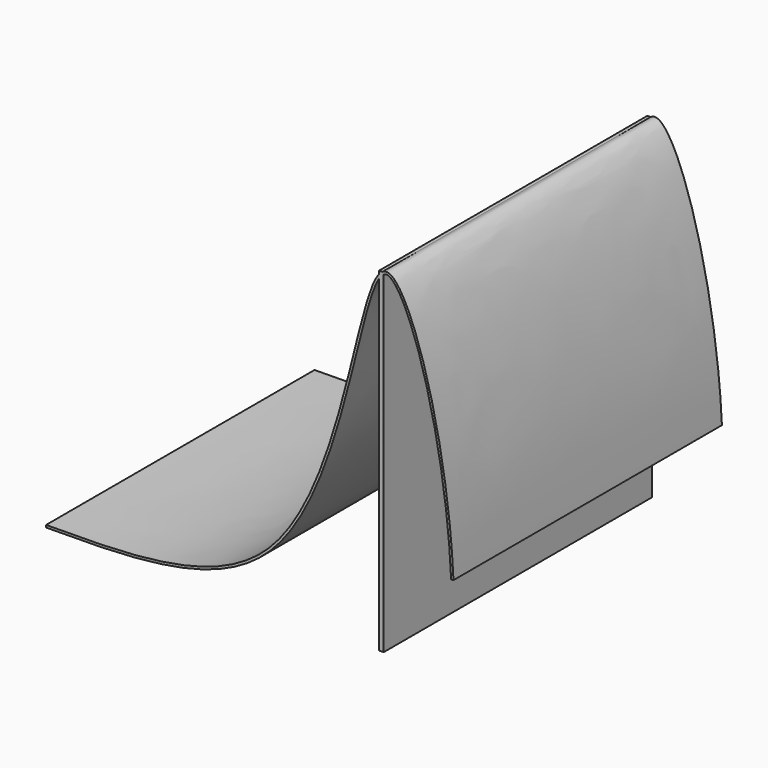
from build123d import *

# Parameters (mm, degrees)
F1_DEPTH = 914.4


# Not quite as in the source:
# - ends of sketch curves that miss each other by under 0.0002 mm in the source are joined
# - the dataset's text gives a spline's control points without its knots; the knots are read off the source's solid


with BuildPart() as f1:
    # F0 (on Front) → F1 (new body)
    with BuildSketch(Plane.XZ):
        with BuildLine():
            add(Edge.make_bspline(
                [(-919.8371731596, 0), (-666.6549326545, 0), (-224.5771125372, 9.857256005), (-90.4120834618, 673.3494347676), (-31.042313376, 873.5728945456), (-12.7, 896.4040661924)],
                knots=[0, 0, 0, 0, 0.2772976129, 0.5617641499, 0.6630198034, 0.6630198034, 0.6630198034, 0.6630198034], degree=3))
            Line((-919.8371731596, 0), (-919.8371731596, -6.35))
            add(Edge.make_bspline(
                [(-919.8371731596, -6.35), (-891.2956817484, -6.35), (-835.0727771699, -6.2264734906), (-753.6955894076, -4.5537616294), (-675.6488494754, -0.2717047035), (-601.3027865804, 7.749478894), (-531.0281070337, 20.6510983897), (-476.1747806697, 36.433071437), (-434.7209643178, 52.6606822547), (-404.9003603349, 66.7779757198), (-376.407262262, 82.9857781471), (-353.8198862803, 98.3520654174), (-336.4752851305, 111.8293289531), (-323.8373430454, 122.5464690045), (-311.5775291009, 133.8876328292), (-299.7039715139, 145.875207016), (-288.2290876414, 158.4866993511), (-273.4422137623, 176.0875345027), (-255.8954652009, 199.4854636313), (-236.2518066429, 229.5516028845), (-211.8312721359, 271.9684188112), (-184.4187186541, 328.7539699263), (-155.8635982627, 401.0055012331), (-131.028728694, 475.4527935567), (-109.3069067738, 550.1778688522), (-90.0991494945, 623.2560938642), (-75.6932560314, 681.1724555189), (-64.8354875196, 724.7427710564), (-56.9528674516, 755.7967634626), (-49.2605256897, 784.9693353051), (-41.6751107234, 811.8671692139), (-34.1167291745, 836.1005454151), (-26.516271345, 857.2638545274), (-20.1072029881, 871.9856586334), (-15.4866518, 880.7508103168), (-13.4472817504, 884.1799958005), (-12.7, 885.3770727094)],
                knots=[0, 0, 0, 0, 0.03125, 0.0625, 0.09375, 0.125, 0.15625, 0.1875, 0.203125, 0.21875, 0.234375, 0.25, 0.2578125, 0.265625, 0.2734375, 0.28125, 0.2890625, 0.296875, 0.3125, 0.328125, 0.34375, 0.375, 0.40625, 0.4375, 0.46875, 0.5, 0.53125, 0.546875, 0.5625, 0.578125, 0.59375, 0.609375, 0.625, 0.640625, 0.6484375, 0.6529650593, 0.6529650593, 0.6529650593, 0.6529650593], degree=3))
            Line((-12.7, 885.3770727094), (-12.7, 896.4040661924))
        make_face()
        with BuildLine():
            Line((-12.7, 904.875), (-12.7, 896.4040661924))
            add(Edge.make_bspline(
                [(-12.7, 896.4040661924), (-9.8289625515, 899.9777238573), (-6.8903732232, 902.823006869), (-3.8687211654, 904.875)],
                knots=[0.6630198034, 0.6630198034, 0.6630198034, 0.6630198034, 0.6788688824, 0.6788688824, 0.6788688824, 0.6788688824], degree=3))
            Line((-3.8687211654, 904.875), (-12.7, 904.875))
        make_face()
        with BuildLine():
            add(Edge.make_bspline(
                [(-12.7, 896.4040661924), (-9.8289625515, 899.9777238573), (-6.8903732232, 902.823006869), (-3.8687211654, 904.875)],
                knots=[0.6630198034, 0.6630198034, 0.6630198034, 0.6630198034, 0.6788688824, 0.6788688824, 0.6788688824, 0.6788688824], degree=3))
            Line((-12.7, 896.4040661924), (-12.7, 885.3770727094))
            add(Edge.make_bspline(
                [(-12.7, 885.3770727094), (-12.1578146641, 886.2456039503), (-10.327872538, 889.0711046998), (-7.2271290281, 893.2451337506), (-3.4946018732, 897.2220843222), (-1.1289437839, 899.0829033781), (0, 899.8227670823)],
                knots=[0.6529650593, 0.6529650593, 0.6529650593, 0.6529650593, 0.65625, 0.6640625, 0.671875, 0.6795490215, 0.6795490215, 0.6795490215, 0.6795490215], degree=3))
            Line((0, 899.8227670823), (0, 904.875))
            Line((0, 904.875), (-3.8687211654, 904.875))
        make_face()
        with BuildLine():
            add(Edge.make_bspline(
                [(-3.8687211654, 904.875), (1.3768159503, 908.437225539), (65.5226358054, 922.1110182588), (174.8235935542, 563.8420495299), (190.3721604559, 228.5401790035)],
                knots=[0.6788688824, 0.6788688824, 0.6788688824, 0.6788688824, 0.7063826167, 1, 1, 1, 1], degree=3))
            Line((-3.8687211654, 904.875), (0, 904.875))
            Line((0, 904.875), (0, 899.8227670823))
            add(Edge.make_bspline(
                [(0, 899.8227670823), (0.0203719127, 899.8361180029), (1.1892498099, 900.5992765813), (2.8626228855, 901.4459342147), (4.9475578198, 902.0833471344), (6.4810971063, 902.345982062), (8.0248389444, 902.405514015), (9.6278327514, 902.2568516663), (11.3272360125, 901.8789926921), (13.1685034705, 901.2342275997), (15.1549787651, 900.2947169392), (17.9792683036, 898.6261359239), (21.7996798698, 895.7330053245), (26.7252350861, 890.9564075118), (31.9010627331, 884.9081499112), (37.2647559638, 877.6325543579), (42.7721833661, 869.1760396376), (50.2634852549, 856.3857689099), (59.838484806, 837.6652789081), (71.5008754365, 811.1500097706), (83.2006513672, 780.8859268301), (94.8138420689, 747.1647527149), (110.0254840172, 697.9743051355), (128.2408613675, 629.2627330137), (147.9185624169, 537.4831514486), (164.5248766535, 438.5937295745), (177.1736880039, 334.8050437488), (182.3793905406, 263.8190463883), (184.0289768201, 228.246033865)],
                knots=[0.6795490215, 0.6795490215, 0.6795490215, 0.6795490215, 0.6796875, 0.6875, 0.69140625, 0.6953125, 0.69921875, 0.703125, 0.70703125, 0.7109375, 0.71484375, 0.71875, 0.7265625, 0.734375, 0.7421875, 0.75, 0.7578125, 0.765625, 0.78125, 0.796875, 0.8125, 0.828125, 0.84375, 0.875, 0.90625, 0.9375, 0.96875, 1, 1, 1, 1], degree=3))
            Line((184.0289768201, 228.246033865), (190.3721604559, 228.5401790035))
        make_face()
        with BuildLine():
            add(Edge.make_bspline(
                [(-12.7, 885.3770727094), (-12.1578146641, 886.2456039503), (-10.327872538, 889.0711046998), (-7.2271290281, 893.2451337506), (-3.4946018732, 897.2220843222), (-1.1289437839, 899.0829033781), (0, 899.8227670823)],
                knots=[0.6529650593, 0.6529650593, 0.6529650593, 0.6529650593, 0.65625, 0.6640625, 0.671875, 0.6795490215, 0.6795490215, 0.6795490215, 0.6795490215], degree=3))
            Line((-12.7, 885.3770727094), (-12.7, -6.35))
            Line((-12.7, -6.35), (0, -6.35))
            Line((0, -6.35), (0, 899.8227670823))
        make_face()
    extrude(amount=F1_DEPTH)


solid = f1.part
